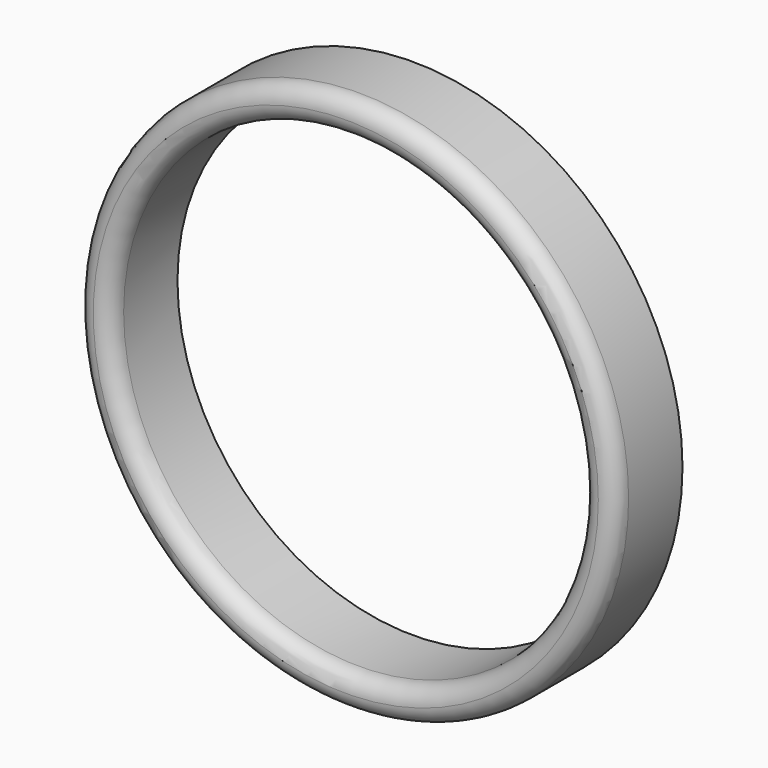
from build123d import *

# Parameters (mm, degrees)
F0_R     = 50.8
F1_DEPTH = 15.875
F2_R     = 44.45
F3_DEPTH = 15.876
F4_R     = 3.17499


# Not quite as in the source:
# - a fillet or chamfer is up to 0.001 mm smaller than in the source, because OpenCascade refuses the exact size


with BuildPart() as f1:
    # F0 (on Front) → F1 (new body)
    with BuildSketch(Plane.XZ):
        Circle(F0_R)
    extrude(amount=F1_DEPTH)

    # F2 (on Front) → F3 (cut, through all)
    with BuildSketch(Plane.XZ):
        Circle(F2_R)
    extrude(amount=F3_DEPTH, mode=Mode.SUBTRACT)

    # F4 (radius 3.175 in the source; OpenCascade refuses exactly that, so slightly less here)
    f4_edges = [f1.edges().sort_by_distance(p)[0] for p in [
        (-50.8, -15.875, 0),
        (-44.45, -15.875, 0),
    ]]
    fillet(f4_edges, radius=F4_R)


solid = f1.part
